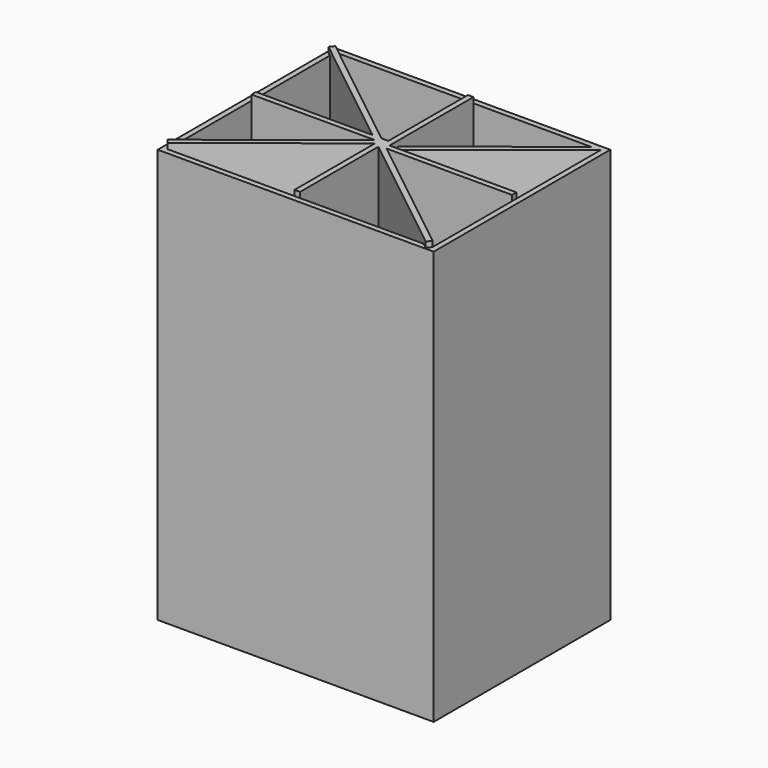
from build123d import *

# Parameters (mm, degrees)
F0_W      = 127
F0_H      = 101.6
F1_DEPTH  = 190.5
F2_T      = -2.54
F10_E18_W = 60.96
F10_E18_H = 190.5
F19_DEPTH = 2.54
F12_E19_W = 77.7505575543
F12_E19_H = 190.5
F20_DEPTH = 2.54
F14_E20_W = 48.26
F14_E20_H = 190.5
F21_DEPTH = 2.54
F16_E21_W = 77.7505575543
F16_E21_H = 190.5
F22_DEPTH = 2.54
F18_E22_W = 60.96
F18_E22_H = 190.5
F23_DEPTH = 2.54
F4_E9_W   = 77.7505575543
F4_E9_H   = 187.96
F24_DEPTH = 2.54
F6_E16_W  = 48.26
F6_E16_H  = 190.5
F25_DEPTH = 2.54
F8_E17_W  = 77.7505575543
F8_E17_H  = 190.5
F26_DEPTH = 2.54


with BuildPart() as f1:
    # F0 (on Top) → F1 (new body)
    with BuildSketch(Plane.XY):
        Rectangle(F0_W, F0_H)
    extrude(amount=F1_DEPTH)

    # F2
    f2_openings = [f1.faces().sort_by_distance(p)[0] for p in [
        (0, 0, 190.5),
    ]]
    offset(amount=F2_T, openings=f2_openings)

    # F10_E18 (on explicit) → F19 (join)
    with BuildSketch(Plane(origin=(0, 0, 2.54), x_dir=(-1, 0, 0), z_dir=(0, 1, 0))):
        with Locations((30.48, 95.25)):
            Rectangle(F10_E18_W, F10_E18_H)
    extrude(amount=F19_DEPTH)

    # F12_E19 (on explicit) → F20 (join)
    with BuildSketch(Plane(origin=(0, 0, 2.54), x_dir=(-0.7840458245, -0.6207029444, 0), z_dir=(-0.6207029444, 0.7840458245, 0))):
        with Locations((38.8752787771, 95.25)):
            Rectangle(F12_E19_W, F12_E19_H)
    extrude(amount=F20_DEPTH)

    # F14_E20 (on explicit) → F21 (join)
    with BuildSketch(Plane(origin=(0, 0, 2.54), x_dir=(0, -1, 0), z_dir=(-1, 0, 0))):
        with Locations((24.13, 95.25)):
            Rectangle(F14_E20_W, F14_E20_H)
    extrude(amount=F21_DEPTH)

    # F16_E21 (on explicit) → F22 (join)
    with BuildSketch(Plane(origin=(0, 0, 2.54), x_dir=(0.7840458245, -0.6207029444, 0), z_dir=(-0.6207029444, -0.7840458245, 0))):
        with Locations((38.8752787771, 95.25)):
            Rectangle(F16_E21_W, F16_E21_H)
    extrude(amount=F22_DEPTH)

    # F18_E22 (on explicit) → F23 (join)
    with BuildSketch(Plane(origin=(0, 0, 2.54), x_dir=(1, 0, 0), z_dir=(0, -1, 0))):
        with Locations((30.48, 95.25)):
            Rectangle(F18_E22_W, F18_E22_H)
    extrude(amount=F23_DEPTH)

    # F4_E9 (on explicit) → F24 (join)
    with BuildSketch(Plane(origin=(60.96, 48.26, 2.54), x_dir=(-0.7840458245, -0.6207029444, 0), z_dir=(-0.6207029444, 0.7840458245, 0))):
        with Locations((38.8752787771, 93.98)):
            Rectangle(F4_E9_W, F4_E9_H)
    extrude(amount=F24_DEPTH)

    # F6_E16 (on explicit) → F25 (join)
    with BuildSketch(Plane(origin=(0, 0, 2.54), x_dir=(0, 1, 0), z_dir=(1, 0, 0))):
        with Locations((24.13, 95.25)):
            Rectangle(F6_E16_W, F6_E16_H)
    extrude(amount=F25_DEPTH)

    # F8_E17 (on explicit) → F26 (join)
    with BuildSketch(Plane(origin=(-60.96, 48.26, 2.54), x_dir=(0.7840458245, -0.6207029444, 0), z_dir=(-0.6207029444, -0.7840458245, 0))):
        with Locations((38.8752787771, 95.25)):
            Rectangle(F8_E17_W, F8_E17_H)
    extrude(amount=F26_DEPTH)


solid = f1.part
